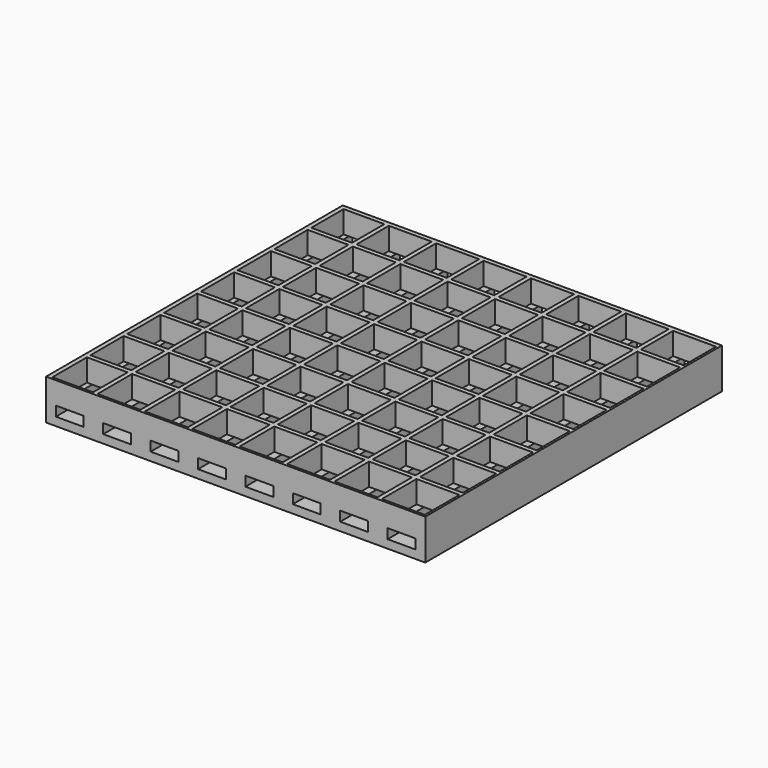
from build123d import *

# Parameters (mm, degrees)
F0_W                 = 3.5
F0_H                 = 3.5
F0_W_2               = 7
F1_DEPTH             = 133
F2_W                 = 1.6
F2_H                 = 8
F2_W_2               = 0.8
F3_DEPTH             = 133
F4_W                 = 1.6
F4_H                 = 8
F4_W_2               = 0.8
F5_DEPTH             = 136
F8_D                 = 3.5
F8_DEPTH             = 12
F8_CSINK_D           = 6.5
F8_CSINK_ANGLE       = 90
F8_TIP               = 1.0515060833
F8_ON_F6_D           = 3.5
F8_ON_F6_DEPTH       = 12
F8_ON_F6_CSINK_D     = 6.5
F8_ON_F6_CSINK_ANGLE = 90
F8_ON_F6_TIP         = 1.0515060833


# Not quite as in the source:
# - a feature names something its author has since deleted; it is built from what else it names


with BuildPart() as f1:
    # F0 (on Front) → F1 (new body)
    with BuildSketch(Plane.XZ):
        with Locations((-66.25, 4.75)):
            Rectangle(F0_W, F0_H)
        with Locations((-17, 4.75)):
            Rectangle(F0_W_2, F0_H)
        with Locations((66.25, 4.75)):
            Rectangle(F0_W, F0_H)
        Polygon((-64.5, 3), (-68, 3), (-68, 0), (68, 0), (68, 3), (64.5, 3), (54.5, 3), (47.5, 3), (37.5, 3), (30.5, 3), (20.5, 3), (13.5, 3), (3.5, 3), (-3.5, 3), (-13.5, 3), (-20.5, 3), (-30.5, 3), (-37.5, 3), (-47.5, 3), (-54.5, 3), align=None)
        with Locations((-51, 4.75)):
            Rectangle(F0_W_2, F0_H)
        with Locations((-34, 4.75)):
            Rectangle(F0_W_2, F0_H)
        with Locations((0, 4.75)):
            Rectangle(F0_W_2, F0_H)
        with Locations((17, 4.75)):
            Rectangle(F0_W_2, F0_H)
        with Locations((34, 4.75)):
            Rectangle(F0_W_2, F0_H)
        with Locations((51, 4.75)):
            Rectangle(F0_W_2, F0_H)
    extrude(amount=F1_DEPTH)

    # F2 (on face) → F3 (join, through all)
    with BuildSketch(Plane.XZ.offset(133)):
        with Locations((-67.2, 10.5)):
            Rectangle(F2_W, F2_H)
        with Locations((-51, 10.5)):
            Rectangle(F2_W, F2_H)
        with Locations((-34, 10.5)):
            Rectangle(F2_W, F2_H)
        with Locations((-17, 10.5)):
            Rectangle(F2_W, F2_H)
        with Locations((0, 10.5)):
            Rectangle(F2_W, F2_H)
        with Locations((17, 10.5)):
            Rectangle(F2_W, F2_H)
        with Locations((34, 10.5)):
            Rectangle(F2_W, F2_H)
        with Locations((51, 10.5)):
            Rectangle(F2_W, F2_H)
        with Locations((67.6, 10.5)):
            Rectangle(F2_W_2, F2_H)
    extrude(amount=-F3_DEPTH)

    # F4 (on face) → F5 (join, through all)
    with BuildSketch(Plane(origin=(-68, 0, 0), x_dir=(0, -1, 0), z_dir=(-1, 0, 0))):
        with Locations((0.8, 10.5)):
            Rectangle(F4_W, F4_H)
        with Locations((16.9, 10.5)):
            Rectangle(F4_W, F4_H)
        with Locations((33.4, 10.5)):
            Rectangle(F4_W, F4_H)
        with Locations((49.9, 10.5)):
            Rectangle(F4_W, F4_H)
        with Locations((66.4, 10.5)):
            Rectangle(F4_W, F4_H)
        with Locations((82.9, 10.5)):
            Rectangle(F4_W, F4_H)
        with Locations((99.4, 10.5)):
            Rectangle(F4_W, F4_H)
        with Locations((115.9, 10.5)):
            Rectangle(F4_W, F4_H)
        with Locations((132.6, 10.5)):
            Rectangle(F4_W_2, F4_H)
    extrude(amount=-F5_DEPTH)

    # F8
    with Locations(Plane.XY.offset(3)):
        with Locations((42.5, -42), (42.5, -91)):
            CounterSinkHole(F8_D / 2, F8_CSINK_D / 2, depth=F8_DEPTH, counter_sink_angle=F8_CSINK_ANGLE)
            with Locations((0, 0, -(F8_DEPTH + F8_TIP / 2))):  # 118° drill point
                Cone(0, F8_D / 2, F8_TIP, mode=Mode.SUBTRACT)

    # F8 on F6
    with Locations(Plane.XY.offset(3)):
        with Locations((-42.5, -42), (-42.5, -91)):
            CounterSinkHole(F8_ON_F6_D / 2, F8_ON_F6_CSINK_D / 2, depth=F8_ON_F6_DEPTH, counter_sink_angle=F8_ON_F6_CSINK_ANGLE)
            with Locations((0, 0, -(F8_ON_F6_DEPTH + F8_ON_F6_TIP / 2))):  # 118° drill point
                Cone(0, F8_ON_F6_D / 2, F8_ON_F6_TIP, mode=Mode.SUBTRACT)


solid = f1.part
